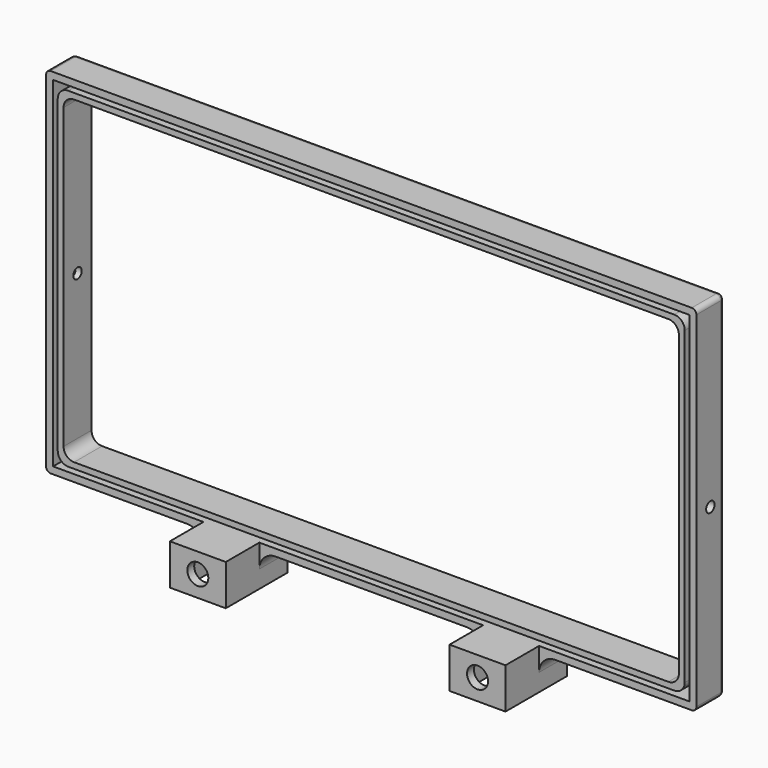
from build123d import *

# Parameters (mm, degrees)
F0_W          = 279
F0_H          = 152
F0_W_2        = 264
F0_H_2        = 137
F1_DEPTH      = 15
F2_W          = 24
F2_H          = 3
F3_DEPTH      = 18
F4_W          = 24
F4_H          = 33
F5_DEPTH      = 14.5
F6_W          = 16.6
F6_H          = 25.6
F7_W          = 16.6
F7_H          = 25.6
F8_DEPTH      = 8.7
F10_R         = 8.3
F9_R          = 8.3
F11_DEPTH     = 25.6
F13_R         = 4.5
F12_R         = 4.5
F14_DEPTH     = 33.001
F15_W         = 273
F15_H         = 146
F15_W_2       = 269
F15_H_2       = 142
F16_DEPTH     = 10
F17_R         = 1.5
F18_DEPTH     = 6
F19_R         = 1.5
F20_DEPTH     = 6
F21_R         = 2
F22_R         = 2.25
F23_DEPTH     = 279.001
F24_R         = 4.5
F25_T1_DEPTH  = 13
F25_T6_ANGLE  = 359.64
F25_T12_ANGLE = 359.64
F25_T18_ANGLE = 359.64
F25_T24_ANGLE = 359.64
F26_R         = 2.5
F27_DEPTH     = 1
F28_R         = 2.5
F29_DEPTH     = 1.5


# Not quite as in the source:
# - a fillet or chamfer that OpenCascade refuses, or shapes differently, is made with other operations: its cross-section is extruded or revolved along the edge and cut away or added


with BuildPart() as f1:
    # F0 (on Front) → F1 (new body)
    with BuildSketch(Plane.XZ):
        Rectangle(F0_W, F0_H)
        Rectangle(F0_W_2, F0_H_2, mode=Mode.SUBTRACT)
    extrude(amount=F1_DEPTH)

    # F2 (on face) → F3 (join)
    with BuildSketch(Plane.XZ.offset(15)):
        with Locations((-60, -74.5)):
            Rectangle(F2_W, F2_H)
        with Locations((60, -74.5)):
            Rectangle(F2_W, F2_H)
    extrude(amount=F3_DEPTH)

    # F4 (on face) → F5 (join)
    with BuildSketch(Plane(origin=(0, 0, -76), x_dir=(1, 0, 0), z_dir=(0, 0, -1))):
        with Locations((-60, 16.5)):
            Rectangle(F4_W, F4_H)
        with Locations((60, 16.5)):
            Rectangle(F4_W, F4_H)
    extrude(amount=F5_DEPTH)

    # F6 (on face) + F7 (on face) → F8 (cut)
    with BuildSketch(Plane(origin=(0, 0, -90.5), x_dir=(1, 0, 0), z_dir=(0, 0, -1))):
        with Locations((-60, 16.5)):
            Rectangle(F6_W, F6_H)
    with BuildSketch(Plane(origin=(0, 0, -90.5), x_dir=(1, 0, 0), z_dir=(0, 0, -1))):
        with Locations((60, 16.5)):
            Rectangle(F7_W, F7_H)
    extrude(amount=-F8_DEPTH, mode=Mode.SUBTRACT)

    # F10 (on face) + F9 (on face) → F11 (cut)
    with BuildSketch(Plane.XZ.offset(3.7)):
        with Locations((60, -81.8)):
            Circle(F10_R)
    with BuildSketch(Plane.XZ.offset(3.7)):
        with Locations((-60, -81.8)):
            Circle(F9_R)
    extrude(amount=F11_DEPTH, mode=Mode.SUBTRACT)

    # F13 (on face) + F12 (on face) → F14 (cut, through all)
    with BuildSketch(Plane.XZ.offset(33)):
        with Locations((60, -81.5)):
            Circle(F13_R)
    with BuildSketch(Plane.XZ.offset(33)):
        with Locations((-60, -81.5)):
            Circle(F12_R)
    extrude(amount=-F14_DEPTH, mode=Mode.SUBTRACT)

    # F15 (on face) → F16 (cut)
    with BuildSketch(Plane.XZ.offset(15)):
        Rectangle(F15_W, F15_H)
        Rectangle(F15_W_2, F15_H_2, mode=Mode.SUBTRACT)
    extrude(amount=-F16_DEPTH, mode=Mode.SUBTRACT)

    # F17 (on face) → F18 (cut)
    with BuildSketch(Plane(origin=(0, 0, -76), x_dir=(1, 0, 0), z_dir=(0, 0, -1))):
        with Locations((-25, 10)):
            Circle(F17_R)
        with Locations((25, 10)):
            Circle(F17_R)
    extrude(amount=-F18_DEPTH, mode=Mode.SUBTRACT)

    # F19 (on face) → F20 (cut)
    with BuildSketch(Plane(origin=(0, 0, 68.5), x_dir=(1, 0, 0), z_dir=(0, 0, -1))):
        with Locations((-122, 10)):
            Circle(F19_R)
        with Locations((122, 10)):
            Circle(F19_R)
    extrude(amount=-F20_DEPTH, mode=Mode.SUBTRACT)

    # F21
    f21_edges = [f1.edges().sort_by_distance(p)[0] for p in [
        (-139.5, 0, 0),
        (-139.5, -7.5, 76),
        (0, 0, 76),
        (-139.5, -7.5, -76),
        (-105.75, 0, -76),
        (0, 0, -76),
        (105.75, 0, -76),
        (139.5, -7.5, -76),
        (139.5, 0, 0),
        (139.5, -7.5, 76),
    ]]
    fillet(f21_edges, radius=F21_R)

    # F22 (on face) → F23 (cut, through all)
    with BuildSketch(Plane(origin=(-139.5, 0, 0), x_dir=(0, -1, 0), z_dir=(-1, 0, 0))):
        with Locations((7.5, -1.62)):
            Circle(F22_R)
    extrude(amount=-F23_DEPTH, mode=Mode.SUBTRACT)

    # F24
    f24_edges = [f1.edges().sort_by_distance(p)[0] for p in [
        (-132, -7.5, 68.5),
        (-134.5, -10, 71),
        (-132, -7.5, -68.5),
        (-134.5, -10, -71),
        (132, -7.5, 68.5),
        (134.5, -10, -71),
        (132, -7.5, -68.5),
        (134.5, -10, 71),
    ]]
    fillet(f24_edges, radius=F24_R)

    # F25: fillet of radius 7 on 4 edges, made by hand

    # F25_s2 → F25_t1 (join)
    with BuildSketch(Plane.XZ.offset(2)):
        with BuildLine():
            ThreePointArc((-72, -83), (-74.0502525317, -78.0502525317), (-79, -76))
            Line((-79, -76), (-72, -76))
            Line((-72, -76), (-72, -83))
        make_face()
        with BuildLine():
            ThreePointArc((48, -83), (45.9497474683, -78.0502525317), (41, -76))
            Line((41, -76), (48, -76))
            Line((48, -76), (48, -83))
        make_face()
        with BuildLine():
            ThreePointArc((72, -83), (74.0502525317, -78.0502525317), (79, -76))
            Line((79, -76), (72, -76))
            Line((72, -76), (72, -83))
        make_face()
        with BuildLine():
            ThreePointArc((-48, -83), (-45.9497474683, -78.0502525317), (-41, -76))
            Line((-41, -76), (-48, -76))
            Line((-48, -76), (-48, -83))
        make_face()
    extrude(amount=F25_T1_DEPTH)


with BuildPart() as f25_tool4:
    # F25_s5 → F25_t6 (revolve)
    with BuildSketch(Plane(origin=(0, -1.5349775685, 0.0096446754), x_dir=(1, 0, 0), z_dir=(0, 0.9999802609, -0.006283144))):
        with BuildLine():
            ThreePointArc((-48, 83.0111055913), (-45.9497474683, 78.061358123), (-41, 76.0111055913))
            Line((-41, 76.0111055913), (-48, 76.0111055913))
            Line((-48, 76.0111055913), (-48, 83.0111055913))
        make_face()
    revolve(axis=Axis((-48, -2, -74), (-1, 0, 0)), revolution_arc=F25_T6_ANGLE)

    split(bisect_by=Plane.XZ, keep=Keep.TOP)

    split(bisect_by=Plane.XY.offset(-73), keep=Keep.BOTTOM)


with BuildPart() as f1_1:
    add(f1.part)

    # F25_t3: union F25_tool4
    add(f25_tool4.part)


with BuildPart() as f25_tool10:
    # F25_s11 → F25_t12 (revolve)
    with BuildSketch(Plane(origin=(0, -1.5349775685, 0.0096446754), x_dir=(1, 0, 0), z_dir=(0, 0.9999802609, -0.006283144))):
        with BuildLine():
            ThreePointArc((72, 83.0111055913), (74.0502525317, 78.061358123), (79, 76.0111055913))
            Line((79, 76.0111055913), (72, 76.0111055913))
            Line((72, 76.0111055913), (72, 83.0111055913))
        make_face()
    revolve(axis=Axis((72, -2, -74), (-1, 0, 0)), revolution_arc=F25_T12_ANGLE)

    split(bisect_by=Plane.XZ, keep=Keep.TOP)

    split(bisect_by=Plane.XY.offset(-73), keep=Keep.BOTTOM)


with BuildPart() as f1_2:
    add(f1_1.part)

    # F25_t9: union F25_tool10
    add(f25_tool10.part)


with BuildPart() as f25_tool16:
    # F25_s17 → F25_t18 (revolve)
    with BuildSketch(Plane(origin=(0, -1.5349775685, 0.0096446754), x_dir=(1, 0, 0), z_dir=(0, 0.9999802609, -0.006283144))):
        with BuildLine():
            ThreePointArc((41, 76.0111055913), (45.9497474683, 78.061358123), (48, 83.0111055913))
            Line((48, 83.0111055913), (48, 76.0111055913))
            Line((48, 76.0111055913), (41, 76.0111055913))
        make_face()
    revolve(axis=Axis((48, -2, -74), (-1, 0, 0)), revolution_arc=F25_T18_ANGLE)

    split(bisect_by=Plane.XZ, keep=Keep.TOP)

    split(bisect_by=Plane.XY.offset(-73), keep=Keep.BOTTOM)


with BuildPart() as f1_3:
    add(f1_2.part)

    # F25_t15: union F25_tool16
    add(f25_tool16.part)


with BuildPart() as f25_tool22:
    # F25_s23 → F25_t24 (revolve)
    with BuildSketch(Plane.XZ.offset(2)):
        with BuildLine():
            ThreePointArc((-72, -83), (-74.0502525317, -78.0502525317), (-79, -76))
            Line((-79, -76), (-72, -76))
            Line((-72, -76), (-72, -83))
        make_face()
    revolve(axis=Axis((-72, -2, -74), (1, 0, 0)), revolution_arc=F25_T24_ANGLE)

    split(bisect_by=Plane.XZ, keep=Keep.TOP)

    split(bisect_by=Plane.XY.offset(-73), keep=Keep.BOTTOM)


with BuildPart() as f1_4:
    add(f1_3.part)

    # F25_t21: union F25_tool22
    add(f25_tool22.part)

    # F26 (on face) → F27 (cut)
    with BuildSketch(Plane(origin=(0, 0, 68.5), x_dir=(1, 0, 0), z_dir=(0, 0, -1))):
        with Locations((-122, 10)):
            Circle(F26_R)
        with Locations((122, 10)):
            Circle(F26_R)
    extrude(amount=-F27_DEPTH, mode=Mode.SUBTRACT)

    # F28 (on face) → F29 (cut)
    with BuildSketch(Plane(origin=(0, 0, -76), x_dir=(1, 0, 0), z_dir=(0, 0, -1))):
        with Locations((-25, 10)):
            Circle(F28_R)
        with Locations((25, 10)):
            Circle(F28_R)
    extrude(amount=-F29_DEPTH, mode=Mode.SUBTRACT)


solid = f1_4.part
